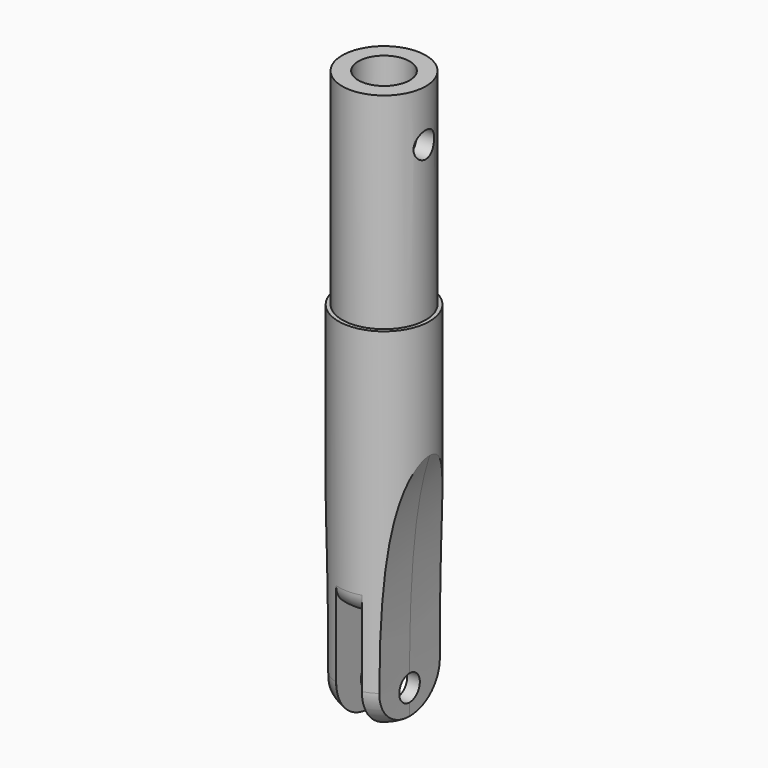
from build123d import *

# Parameters (mm, degrees)
F0_R           = 10.3251
F1_DEPTH       = 50.8
F2_R           = 11.2649
F3_DEPTH       = 88.9
F4_R           = 3.175
F5_DEPTH       = 11.2659
F5_DEPTH_BACK  = 11.2659
F6_W           = 12.7
F6_H           = 12.7
F7_DEPTH       = 11.2659
F7_DEPTH_BACK  = 11.2659
F8_R           = 3.175
F9_DEPTH       = 11.2659001
F9_DEPTH_BACK  = 11.2659001
F10_T2_ANGLE   = 327.0642364541
F10_T4_ANGLE   = 327.0642364541
F11_R          = 6.35
F12_DEPTH      = 76.2
F13_W          = 6.35
F13_H          = 31.75
F14_DEPTH      = 11.2659001
F14_DEPTH_BACK = 11.2659001
F15_R          = 5.08


# Not quite as in the source:
# - a fillet or chamfer that OpenCascade refuses, or shapes differently, is made with other operations: its cross-section is extruded or revolved along the edge and cut away or added


with BuildPart() as f1:
    # F0 (on Top) → F1 (new body)
    with BuildSketch(Plane.XY):
        Circle(F0_R)
    extrude(amount=F1_DEPTH)

    # F2 (on face) → F3 (join)
    with BuildSketch(Plane(origin=(0, 0, 0), x_dir=(1, 0, 0), z_dir=(0, 0, -1))):
        Circle(F2_R)
    extrude(amount=F3_DEPTH)

    # F4 (on Right) → F5 (cut, two sides)
    with BuildSketch(Plane.YZ) as f5_sk:
        with Locations((0, 38.1)):
            Circle(F4_R)
    extrude(amount=-F5_DEPTH, mode=Mode.SUBTRACT)
    extrude(f5_sk.sketch, amount=F5_DEPTH_BACK, mode=Mode.SUBTRACT)

    # F6 (on Front) → F7 (cut, two sides)
    with BuildSketch(Plane.XZ) as f7_sk:
        with Locations((-12.7, -95.25)):
            Rectangle(F6_W, F6_H)
        with BuildLine():
            Line((-19.05, -88.9), (-6.35, -88.9))
            add(Edge.make_bspline(
                [(-12.7, -25.4), (-6.5615815111, -39.3321929336), (-6.1049603775, -64.6134701729), (-6.35, -88.9)],
                knots=[0, 0, 0, 0, 63.8167101941, 63.8167101941, 63.8167101941, 63.8167101941], degree=3))
            Line((-12.7, -25.4), (-19.05, -88.9))
        make_face()
        with BuildLine():
            add(Edge.make_bspline(
                [(12.7, -25.4), (6.5615815111, -39.3321929336), (6.1049603775, -64.6134701729), (6.35, -88.9)],
                knots=[0, 0, 0, 0, 63.8167101941, 63.8167101941, 63.8167101941, 63.8167101941], degree=3))
            Line((6.35, -88.9), (19.05, -88.9))
            Line((19.05, -88.9), (12.7, -25.4))
        make_face()
        with Locations((12.7, -95.25)):
            Rectangle(F6_W, F6_H)
    extrude(amount=-F7_DEPTH, mode=Mode.SUBTRACT)
    extrude(f7_sk.sketch, amount=F7_DEPTH_BACK, mode=Mode.SUBTRACT)

    # F8 (on Right) → F9 (cut, two sides)
    with BuildSketch(Plane.YZ) as f9_sk:
        with Locations((0, -81.28)):
            Circle(F8_R)
    extrude(amount=-F9_DEPTH, mode=Mode.SUBTRACT)
    extrude(f9_sk.sketch, amount=F9_DEPTH_BACK, mode=Mode.SUBTRACT)

    # F10: fillet of radius 10.16 on 2 edges, made by hand

    # F10_s1 → F10_t2 (revolve, cut)
    with BuildSketch(Plane(origin=(0, 0, 0), x_dir=(0, 0, 1), z_dir=(0.9589787944, -0.2834778157, 0))):
        with BuildLine():
            ThreePointArc((-78.74, 11.2649), (-85.9242048969, 8.2891048969), (-88.9, 1.1049))
            Line((-88.9, 1.1049), (-88.9, 11.2649))
            Line((-88.9, 11.2649), (-78.74, 11.2649))
        make_face()
    revolve(axis=Axis((0, 0, -88.9), (0, 0, -1)), revolution_arc=F10_T2_ANGLE, mode=Mode.SUBTRACT)

    # F10_s3 → F10_t4 (revolve, cut)
    with BuildSketch(Plane(origin=(0, 0, 0), x_dir=(0, 0, 1), z_dir=(-0.9589787944, 0.2834778157, 0))):
        with BuildLine():
            ThreePointArc((-78.74, 11.2649), (-85.9242048969, 8.2891048969), (-88.9, 1.1049))
            Line((-88.9, 1.1049), (-88.9, 11.2649))
            Line((-88.9, 11.2649), (-78.74, 11.2649))
        make_face()
    revolve(axis=Axis((0, 0, -88.9), (0, 0, -1)), revolution_arc=F10_T4_ANGLE, mode=Mode.SUBTRACT)

    # F11 (on face) → F12 (cut)
    with BuildSketch(Plane.XY.offset(50.8)):
        Circle(F11_R)
    extrude(amount=-F12_DEPTH, mode=Mode.SUBTRACT)

    # F13 (on Front) → F14 (cut, two sides)
    with BuildSketch(Plane.XZ) as f14_sk:
        with Locations((0, -78.74)):
            Rectangle(F13_W, F13_H)
    extrude(amount=-F14_DEPTH, mode=Mode.SUBTRACT)
    extrude(f14_sk.sketch, amount=F14_DEPTH_BACK, mode=Mode.SUBTRACT)

    # F15
    f15_edges = [f1.edges().sort_by_distance(p)[0] for p in [
        (0, 11.2649, -62.865),
        (0, -11.2649, -62.865),
    ]]
    fillet(f15_edges, radius=F15_R)


solid = f1.part
